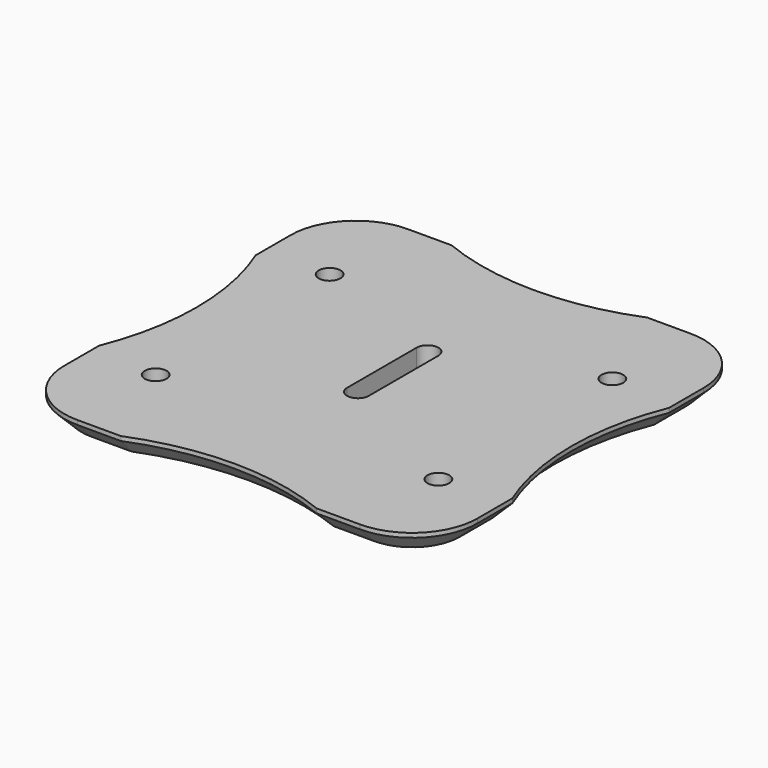
from build123d import *

# Parameters (mm, degrees)
F0_W     = 120.65
F0_H     = 120.65
F0_R     = 3.175
F1_DEPTH = 6.35
F4_DEPTH = 25.4
F5_R     = 3.175
F6_DEPTH = 25.4
F7_SIZE  = 5.08


# Not quite as in the source:
# - a feature of the source that left no trace in its solid (it failed there, or was rolled back) is left out


with BuildPart() as f1:
    # F0 (on Top) → F1 (new body)
    with BuildSketch(Plane.XY):
        Rectangle(F0_W, F0_H)
        with Locations((-41.275, -31.75)):
            Circle(F0_R, mode=Mode.SUBTRACT)
        with Locations((41.275, -31.75)):
            Circle(F0_R, mode=Mode.SUBTRACT)
        with Locations((-41.275, 31.75)):
            Circle(F0_R, mode=Mode.SUBTRACT)
        with Locations((41.275, 31.75)):
            Circle(F0_R, mode=Mode.SUBTRACT)
    extrude(amount=F1_DEPTH)

    # F2 (on face) → F4 (cut)
    with BuildSketch(Plane(origin=(0, 0, 0), x_dir=(1, 0, 0), z_dir=(0, 0, -1))):
        with BuildLine():
            ThreePointArc((-3.175, -15.875), (0, -19.05), (3.175, -15.875))
            ThreePointArc((3.175, -15.875), (0, -12.7), (-3.175, -15.875))
        make_face()
        with BuildLine():
            ThreePointArc((-3.175, -15.875), (0, -12.7), (3.175, -15.875))
            Line((3.1750000339, -15.875), (3.1713092382, 9.3719551838))
            ThreePointArc((3.1713092382, 9.3719551838), (-0.0765446561, 6.3509228246), (-3.175, 9.525))
            Line((-3.175, 9.525), (-3.175, -15.875))
        make_face()
        with BuildLine():
            Line((3.1712643561, 9.6789720229), (3.1713092382, 9.3719551838))
            ThreePointArc((3.1713092382, 9.3719551838), (3.1740771754, 9.4484553439), (3.175, 9.525))
            ThreePointArc((3.175, 9.525), (3.1740659516, 9.6020086665), (3.1712643561, 9.6789720229))
        make_face()
        with BuildLine():
            ThreePointArc((-3.175, 9.525), (-0.0765446561, 6.3509228246), (3.1713092382, 9.3719551838))
            Line((3.1713092382, 9.3719551838), (3.1712643561, 9.6789720229))
            ThreePointArc((3.1712643561, 9.6789720229), (-0.0770086665, 12.6990659516), (-3.175, 9.525))
        make_face()
    extrude(amount=-F4_DEPTH, mode=Mode.SUBTRACT)

    # F5 (on face) → F6 (cut)
    with BuildSketch(Plane.XY.offset(6.35)):
        with BuildLine():
            ThreePointArc((-28.575, 60.325), (0, 54.7642905896), (28.575, 60.325))
            Line((28.575, 60.325), (-28.575, 60.325))
        make_face()
        with BuildLine():
            Line((-28.575, -60.325), (28.575, -60.325))
            ThreePointArc((28.575, -60.325), (0, -54.7642905896), (-28.575, -60.325))
        make_face()
        with BuildLine():
            Line((60.325, -28.575), (60.325, 28.575))
            ThreePointArc((60.325, 28.575), (54.7642905896, 0), (60.325, -28.575))
        make_face()
        with BuildLine():
            ThreePointArc((-60.325, -28.575), (-54.7642905896, 0), (-60.325, 28.575))
            Line((-60.325, 28.575), (-60.325, -28.575))
        make_face()
        with Locations((41.275, 31.75)):
            Circle(F5_R)
        with Locations((41.275, -31.75)):
            Circle(F5_R)
        with Locations((-41.275, -31.75)):
            Circle(F5_R)
        with Locations((-41.275, 31.75)):
            Circle(F5_R)
        with BuildLine():
            Line((60.325, 60.325), (41.275, 60.325))
            ThreePointArc((41.275, 60.325), (54.7453841816, 54.7453841816), (60.325, 41.275))
            Line((60.325, 41.275), (60.325, 60.325))
        make_face()
        with BuildLine():
            ThreePointArc((-41.275, -60.325), (-54.7453841816, -54.7453841816), (-60.325, -41.275))
            Line((-60.325, -41.275), (-60.325, -60.325))
            Line((-60.325, -60.325), (-41.275, -60.325))
        make_face()
        with BuildLine():
            ThreePointArc((-60.325, 41.275), (-54.7453841816, 54.7453841816), (-41.275, 60.325))
            Line((-41.275, 60.325), (-60.325, 60.325))
            Line((-60.325, 60.325), (-60.325, 41.275))
        make_face()
        with BuildLine():
            Line((60.325, -60.325), (60.325, -41.275))
            ThreePointArc((60.325, -41.275), (54.7453841816, -54.7453841816), (41.275, -60.325))
            Line((41.275, -60.325), (60.325, -60.325))
        make_face()
    extrude(amount=-F6_DEPTH, mode=Mode.SUBTRACT)

    # F7
    f7_edges = [f1.edges().sort_by_distance(p)[0] for p in [
        (0, 54.764291, 0),
        (54.745384, 54.745384, 0),
        (54.764291, 0, 0),
        (54.745384, -54.745384, 0),
        (-34.925, -60.325, 0),
        (0, -54.764291, 0),
        (-54.745384, 54.745384, 0),
        (-60.325, 34.925, 0),
        (-54.764291, 0, 0),
        (-54.745384, -54.745384, 0),
        (-60.325, -34.925, 0),
        (-34.925, 60.325, 0),
        (34.925, 60.325, 0),
        (60.325, 34.925, 0),
        (60.325, -34.925, 0),
        (34.925, -60.325, 0),
    ]]
    chamfer(f7_edges, length=F7_SIZE)


solid = f1.part
